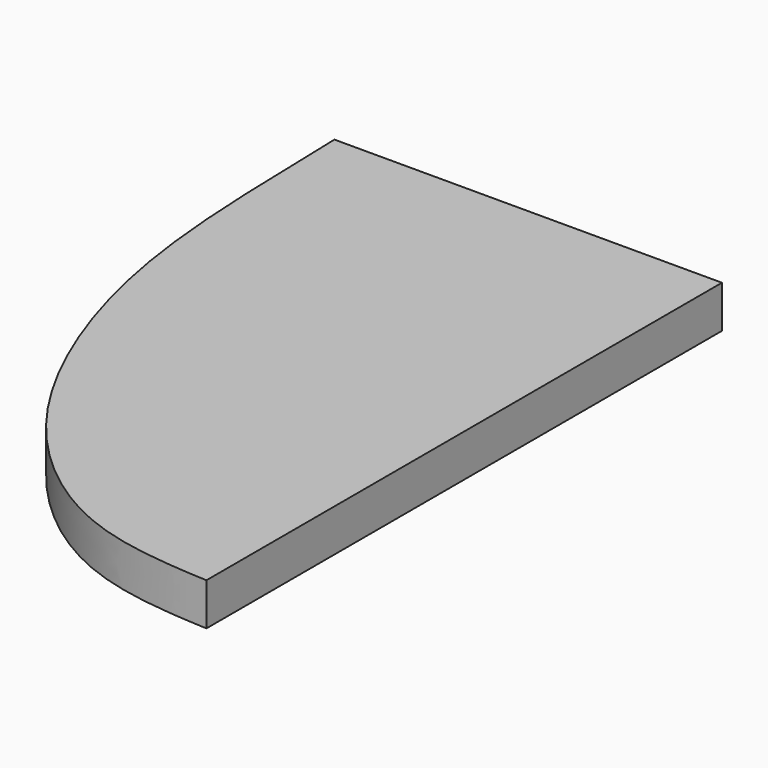
from build123d import *

# Parameters (mm, degrees)
F1_DEPTH = 25


# Not quite as in the source:
# - a feature names something its author has since deleted; it is built from what else it names


with BuildPart() as f1:
    # F0 (on Top) → F1 (new body)
    with BuildSketch(Plane.XY):
        with BuildLine():
            Line((0, 0), (-228.5, 0))
            add(Edge.make_bspline(
                [(-228.5, 0), (-226.8024807913, -61.2307032026), (-226.7186497639, -160.2488878314), (-170.6961741077, -301.5507488185), (-83.1590128355, -374.4708739919), (-26.2308287082, -378.5725320699), (0, -380)],
                knots=[0, 0, 0, 0, 0.2902408691, 0.5636030239, 0.7977729188, 1, 1, 1, 1], degree=3))
            Line((0, -380), (0, 0))
        make_face()
    extrude(amount=F1_DEPTH)


solid = f1.part
